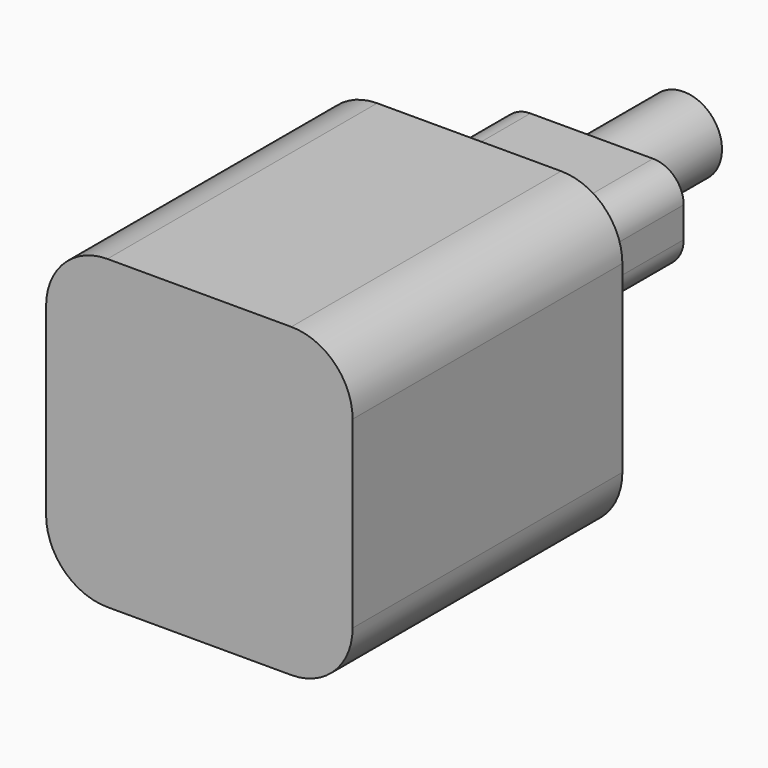
from build123d import *

# Parameters (mm, degrees)
F0_W      = 25.4
F0_H      = 25.4
F1_DEPTH  = 27.94
F2_R      = 5.08
F3_R      = 5.08
F4_R      = 5.08
F5_R      = 5.08
F6_W      = 15.24
F6_H      = 7.62
F7_DEPTH  = 12.7
F8_R      = 2.54
F9_R      = 2.54
F10_R     = 2.54
F11_R     = 2.54
F12_R     = 3.175
F14_DEPTH = 9.525


with BuildPart() as f1:
    # F0 (on Front) → F1 (new body)
    with BuildSketch(Plane.XZ):
        with Locations((12.7, -12.7)):
            Rectangle(F0_W, F0_H)
    extrude(amount=F1_DEPTH)

    # F2
    f2_edges = [f1.edges().sort_by_distance(p)[0] for p in [
        (25.4, -13.97, 0),
    ]]
    fillet(f2_edges, radius=F2_R)

    # F3
    f3_edges = [f1.edges().sort_by_distance(p)[0] for p in [
        (0, -13.97, 0),
    ]]
    fillet(f3_edges, radius=F3_R)

    # F4
    f4_edges = [f1.edges().sort_by_distance(p)[0] for p in [
        (25.4, -13.97, -25.4),
    ]]
    fillet(f4_edges, radius=F4_R)

    # F5
    f5_edges = [f1.edges().sort_by_distance(p)[0] for p in [
        (0, -13.97, -25.4),
    ]]
    fillet(f5_edges, radius=F5_R)

    # F6 (on face) → F7 (join)
    with BuildSketch(Plane(origin=(0, 0, 0), x_dir=(-1, 0, 0), z_dir=(0, 1, 0))):
        with Locations((-12.7, -8.89)):
            Rectangle(F6_W, F6_H)
    extrude(amount=F7_DEPTH)

    # F8
    f8_edges = [f1.edges().sort_by_distance(p)[0] for p in [
        (5.08, 6.35, -5.08),
    ]]
    fillet(f8_edges, radius=F8_R)

    # F9
    f9_edges = [f1.edges().sort_by_distance(p)[0] for p in [
        (5.08, 6.35, -12.7),
    ]]
    fillet(f9_edges, radius=F9_R)

    # F10
    f10_edges = [f1.edges().sort_by_distance(p)[0] for p in [
        (20.32, 6.35, -5.08),
    ]]
    fillet(f10_edges, radius=F10_R)

    # F11
    f11_edges = [f1.edges().sort_by_distance(p)[0] for p in [
        (20.32, 6.35, -12.7),
    ]]
    fillet(f11_edges, radius=F11_R)

    # F12 (on face) → F14 (join)
    with BuildSketch(Plane(origin=(0, 12.7, 0), x_dir=(-1, 0, 0), z_dir=(0, 1, 0))):
        with Locations((-12.7, -8.89)):
            Circle(F12_R)
    extrude(amount=F14_DEPTH)


solid = f1.part
